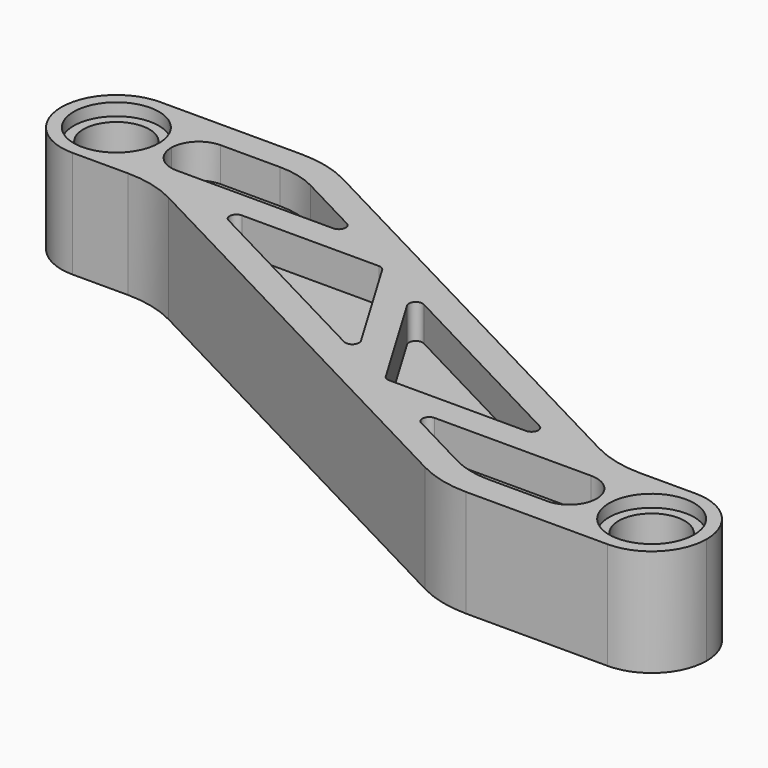
from build123d import *

# Parameters (mm, degrees)
F1_DEPTH  = 3.9
F3_DEPTH  = 2.5
F5_DEPTH  = 2.5
F6_R      = 8
F7_R      = 3.99999
F8_R      = 2.4
F9_DEPTH  = 3.901
F8_R_2    = 3.1
F10_DEPTH = 0.9
F12_R     = 1.99999
F13_R     = 6
F14_R     = 0.5


# Not quite as in the source:
# - a fillet or chamfer is up to 0.001 mm smaller than in the source, because OpenCascade refuses the exact size


with BuildPart() as f1:
    # F0 (on Top) → F1 (new body)
    with BuildSketch(Plane.XY):
        Polygon((-10.2351482974, 8), (-26.5155562797, 8), (-26.5155562797, 0), (-16.5155562797, 0), (19.0857153862, -18.6285724837), (35.3661233686, -18.6285724837), (35.3661233686, -10.6285724837), (25.3661233686, -10.6285724837), align=None)
    extrude(amount=F1_DEPTH)

    # F2 (on face) → F3 (cut)
    with BuildSketch(Plane.XY.offset(3.9)):
        Polygon((24.8744862124, -12.6285724837), (-10.7267854535, 6), (-18.5155562797, 6), (-18.5155562797, 2), (-16.0239191236, 2), (19.5773525424, -16.6285724837), (27.3661233686, -16.6285724837), (27.3661233686, -12.6285724837), align=None)
    extrude(amount=-F3_DEPTH, mode=Mode.SUBTRACT)

    # F4 (on face) → F5 (join, through all)
    with BuildSketch(Plane.XY.offset(3.9)):
        Polygon((11.9329081391, -12.6285724837), (24.8744862124, -12.6285724837), (21.0522640108, -10.6285724837), (8.7555263004, -10.6285724837), (3.1855427267, -1.2797066451), (0.7398811514, 0), (0.0950407885, 0), (5.6650243622, -9.3488658386), align=None)
        Polygon((-12.201696922, 0), (0.0950407885, 0), (-0.1970488953, 0.4902540968), (-3.0823410503, 2), (-16.0239191236, 2), align=None)
        Polygon((-0.1970488953, 0.4902540968), (0.0950407885, 0), (0.7398811514, 0), align=None)
    extrude(amount=-F5_DEPTH)

    # F6
    f6_edges = [f1.edges().sort_by_distance(p)[0] for p in [
        (-10.235148, 8, 1.95),
        (25.366123, -10.628572, 1.95),
        (19.085715, -18.628572, 1.95),
        (-16.515556, 0, 1.95),
    ]]
    fillet(f6_edges, radius=F6_R)

    # F7 (radius 4 in the source; OpenCascade refuses exactly that, so slightly less here)
    f7_edges = [f1.edges().sort_by_distance(p)[0] for p in [
        (-26.515556, 8, 1.95),
        (-26.515556, 0, 1.95),
        (35.366123, -10.628572, 1.95),
        (35.366123, -18.628572, 1.95),
    ]]
    fillet(f7_edges, radius=F7_R)

    # F8 (on face) → F9 (cut, through all)
    with BuildSketch(Plane.XY.offset(3.9)):
        with Locations((-22.5155562797, 4)):
            Circle(F8_R)
        with Locations((31.3661233686, -14.6285724837)):
            Circle(F8_R)
    extrude(amount=-F9_DEPTH, mode=Mode.SUBTRACT)

    # F8 (on face) → F10 (cut)
    with BuildSketch(Plane.XY.offset(3.9)):
        with Locations((-22.5155562797, 4)):
            Circle(F8_R_2)
        with Locations((-22.5155562797, 4)):
            Circle(F8_R, mode=Mode.SUBTRACT)
        with Locations((31.3661233686, -14.6285724837)):
            Circle(F8_R_2)
        with Locations((31.3661233686, -14.6285724837)):
            Circle(F8_R, mode=Mode.SUBTRACT)
    extrude(amount=-F10_DEPTH, mode=Mode.SUBTRACT)

    # F11: F1 across face


with BuildPart() as f1_1:
    add(f1.part)
    add(f1.part.mirror(Plane(origin=(4.4252835444, -5.3142862419, 0), x_dir=(1, 0, 0), z_dir=(0, 0, -1))))

    # F12 (radius 2 in the source; OpenCascade refuses exactly that, so slightly less here)
    f12_edges = [f1_1.edges().sort_by_distance(p)[0] for p in [
        (27.366123, -16.628572, 2.65),
        (27.366123, -12.628572, 2.65),
        (-18.515556, 2, 2.65),
        (-18.515556, 6, 2.65),
        (-18.515556, 2, -2.65),
        (-18.515556, 6, -2.65),
        (27.366123, -16.628572, -2.65),
        (27.366123, -12.628572, -2.65),
    ]]
    fillet(f12_edges, radius=F12_R)

    # F13
    f13_edges = [f1_1.edges().sort_by_distance(p)[0] for p in [
        (19.577353, -16.628572, -2.65),
        (-10.726785, 6, -2.65),
        (-10.726785, 6, 2.65),
        (19.577353, -16.628572, 2.65),
    ]]
    fillet(f13_edges, radius=F13_R)

    # F14
    f14_edges = [f1_1.edges().sort_by_distance(p)[0] for p in [
        (8.755526, -10.628572, 2.65),
        (21.052264, -10.628572, 2.65),
        (3.185543, -1.279707, 2.65),
        (11.932908, -12.628572, 2.65),
        (-12.201697, 0, 2.65),
        (0.095041, 0, 2.65),
        (5.665024, -9.348866, 2.65),
        (-3.082341, 2, 2.65),
        (-3.082341, 2, -2.65),
        (21.052264, -10.628572, -2.65),
        (-12.201697, 0, -2.65),
        (11.932908, -12.628572, -2.65),
        (8.755526, -10.628572, -2.65),
        (3.185543, -1.279707, -2.65),
        (0.095041, 0, -2.65),
        (5.665024, -9.348866, -2.65),
    ]]
    fillet(f14_edges, radius=F14_R)


solid = f1_1.part
